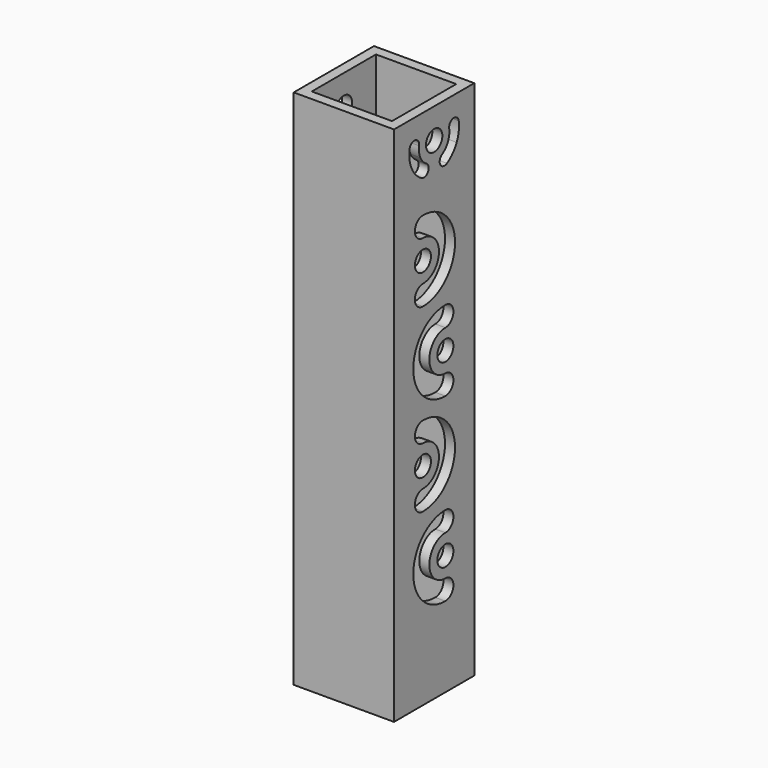
from build123d import *

# Parameters (mm, degrees)
F0_W     = 63.5
F0_H     = 63.5
F0_W_2   = 50.8
F0_H_2   = 50.8
F1_DEPTH = 165.1
F3_R     = 6.477
F4_DEPTH = 25.4
F6_DEPTH = 25.4
F7_R     = 6.35
F8_DEPTH = 63.501


# Not quite as in the source:
# - ends of sketch curves that miss each other by under 0.0002 mm in the source are joined


with BuildPart() as f1:
    # F0 (on Top) → F1 (new body, symmetric)
    with BuildSketch(Plane.XY):
        Rectangle(F0_W, F0_H)
        Rectangle(F0_W_2, F0_H_2, mode=Mode.SUBTRACT)
    extrude(amount=F1_DEPTH, both=True)

    # F3 (on face) → F4 (cut)
    with BuildSketch(Plane.YZ.offset(31.75)):
        with Locations((0, 146.05)):
            Circle(F3_R)
        with BuildLine():
            ThreePointArc((10.1385245046, 129.1766616857), (14.6288058895, 132.8781640138), (17.8406687878, 137.7307595176))
            ThreePointArc((17.8406687878, 137.7307595176), (19.4934269332, 143.3103775076), (19.4426449846, 149.1294124443))
            ThreePointArc((19.4426449846, 149.1294124443), (15.0835370951, 152.2964897102), (11.9164598293, 147.9373818207))
            ThreePointArc((11.9164598293, 147.9373818207), (11.9475842494, 144.3708765369), (10.9346034506, 140.9511106721))
            ThreePointArc((10.9346034506, 140.9511106721), (8.9660423194, 137.9769392343), (6.2139343738, 135.708276517))
            ThreePointArc((6.2139343738, 135.708276517), (4.9104220235, 130.4801740359), (10.1385245046, 129.1766616857))
        make_face()
        with BuildLine():
            ThreePointArc((-10.1385245046, 129.1766616857), (-4.9104220235, 130.4801740359), (-6.2139343738, 135.708276517))
            ThreePointArc((-6.2139343738, 135.708276517), (-8.9660423194, 137.9769392343), (-10.9346034506, 140.9511106721))
            ThreePointArc((-10.9346034506, 140.9511106721), (-11.9475842494, 144.3708765369), (-11.9164598293, 147.9373818207))
            ThreePointArc((-11.9164598293, 147.9373818207), (-15.0835370951, 152.2964897102), (-19.4426449846, 149.1294124443))
            ThreePointArc((-19.4426449846, 149.1294124443), (-19.4934269332, 143.3103775076), (-17.8406687878, 137.7307595176))
            ThreePointArc((-17.8406687878, 137.7307595176), (-14.6288058895, 132.8781640138), (-10.1385245046, 129.1766616857))
        make_face()
    extrude(amount=-F4_DEPTH, mode=Mode.SUBTRACT)

    # F5 (on face) → F6 (cut)
    with BuildSketch(Plane(origin=(-31.75, 0, 0), x_dir=(0, -1, 0), z_dir=(-1, 0, 0))):
        with BuildLine():
            ThreePointArc((-3.1401119103, 140.3850881569), (3.2873259769, 140.4692279278), (6.477, 146.05))
            ThreePointArc((6.477, 146.05), (-3.2873259769, 151.6307720722), (-3.1401119103, 140.3850881569))
        make_face()
        with BuildLine():
            ThreePointArc((-5.7913527214, 132.1654121492), (-6.0549491708, 133.1322727306), (-6.7727903948, 133.8315626913))
            ThreePointArc((-6.7727903948, 133.8315626913), (-9.3377562721, 131.1985515677), (-5.7913527214, 132.1654121492))
        make_face()
        with BuildLine():
            ThreePointArc((3.1226517792, 134.3961049058), (0.4285749428, 129.7298269458), (5.0948529028, 127.0357501095))
            ThreePointArc((5.0948529028, 127.0357501095), (17.8406687878, 137.7307595176), (17.8406687878, 154.3692404824))
            ThreePointArc((17.8406687878, 154.3692404824), (12.777460542, 156.2120975737), (10.9346034506, 151.1488893279))
            ThreePointArc((10.9346034506, 151.1488893279), (10.9346034506, 140.9511106721), (3.1226517792, 134.3961049058))
        make_face()
    extrude(amount=-F6_DEPTH, mode=Mode.SUBTRACT)

    # F7 (on face) → F8 (cut, through all)
    with BuildSketch(Plane.YZ.offset(31.75)):
        with BuildLine():
            ThreePointArc((-8.89, 107.949999693), (-15.239999693, 101.6), (-8.89, 95.250000307))
            ThreePointArc((-8.89, 95.250000307), (3.81, 82.55), (-8.89, 69.85))
            ThreePointArc((-8.89, 69.85), (-15.239999693, 63.5), (-8.89, 57.150000307))
            ThreePointArc((-8.89, 57.150000307), (16.509999693, 82.55), (-8.89, 107.949999693))
        make_face()
        with BuildLine():
            ThreePointArc((8.89, 3.07e-07), (15.239999693, 6.35), (8.89, 12.699999693))
            ThreePointArc((8.89, 12.699999693), (-3.81, 25.4), (8.89, 38.1))
            ThreePointArc((8.89, 38.1), (15.24, 44.45), (8.89, 50.8))
            ThreePointArc((8.89, 50.8), (-16.509999693, 25.4), (8.89, 3.07e-07))
        make_face()
        with BuildLine():
            ThreePointArc((-8.89, -6.350000307), (-15.239999693, -12.7), (-8.89, -19.049999693))
            ThreePointArc((-8.89, -19.049999693), (3.81, -31.75), (-8.89, -44.45))
            ThreePointArc((-8.89, -44.45), (-15.239999693, -50.8), (-8.89, -57.149999693))
            ThreePointArc((-8.89, -57.149999693), (16.509999693, -31.75), (-8.89, -6.350000307))
        make_face()
        with BuildLine():
            ThreePointArc((8.89, -114.299999693), (15.239999693, -107.95), (8.89, -101.600000307))
            ThreePointArc((8.89, -101.600000307), (-3.81, -88.9), (8.89, -76.2))
            ThreePointArc((8.89, -76.2), (15.24, -69.85), (8.89, -63.5))
            ThreePointArc((8.89, -63.5), (-16.509999693, -88.9), (8.89, -114.299999693))
        make_face()
        with Locations((-8.89, 82.55)):
            Circle(F7_R)
        with Locations((8.89, 25.4)):
            Circle(F7_R)
        with Locations((8.89, -88.9)):
            Circle(F7_R)
        with Locations((-8.89, -31.75)):
            Circle(F7_R)
    extrude(amount=-F8_DEPTH, mode=Mode.SUBTRACT)


solid = f1.part
